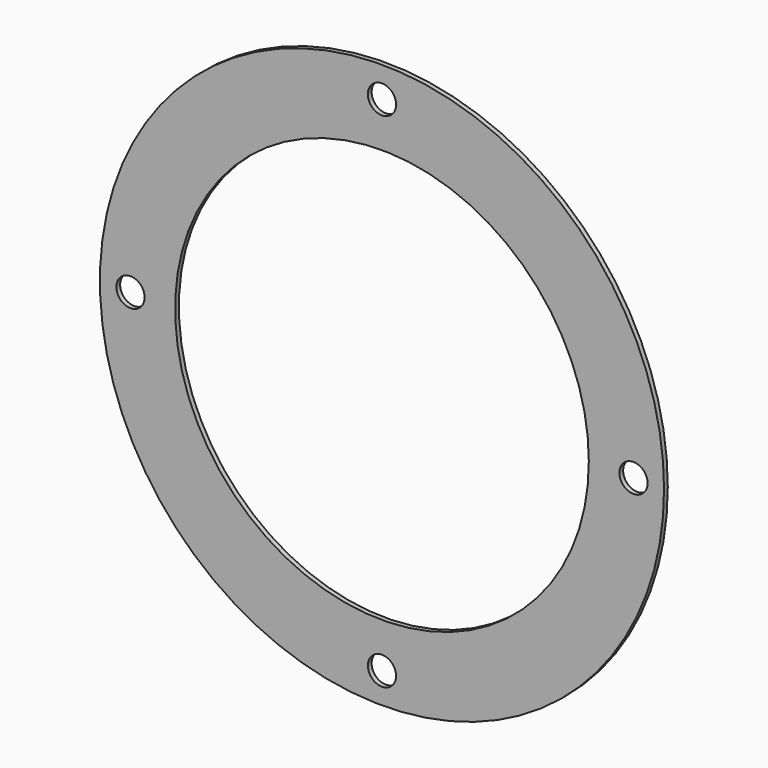
from build123d import *

# Parameters (mm, degrees)
F0_R     = 95.25
F0_R_2   = 4.7625
F0_R_3   = 69.85
F1_DEPTH = 1.5875


# Not quite as in the source:
# - a length typed as a fraction of an inch, garbled in the dataset ("3 / 203.2 mm" for 3/8 in), is restored


with BuildPart() as f1:
    # F0 (on Front) → F1 (new body)
    with BuildSketch(Plane.XZ):
        Circle(F0_R)
        with Locations((0, -84.93125)):
            Circle(F0_R_2, mode=Mode.SUBTRACT)
        with Locations((-84.93125, 0)):
            Circle(F0_R_2, mode=Mode.SUBTRACT)
        Circle(F0_R_3, mode=Mode.SUBTRACT)
        with Locations((84.93125, 0)):
            Circle(F0_R_2, mode=Mode.SUBTRACT)
        with Locations((0, 84.93125)):
            Circle(F0_R_2, mode=Mode.SUBTRACT)
    extrude(amount=F1_DEPTH)


solid = f1.part
